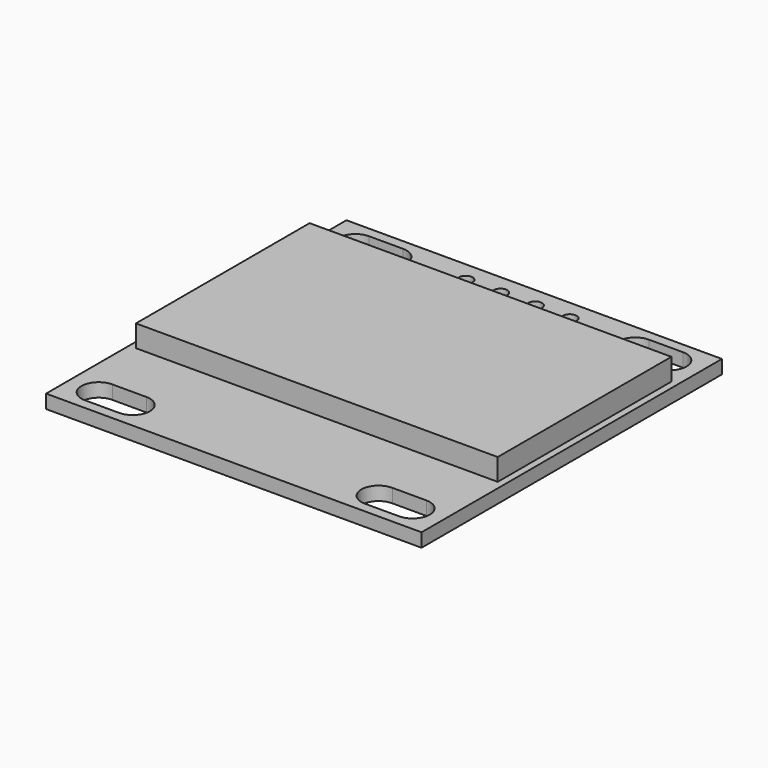
from build123d import *

# Parameters (mm, degrees)
F0_W           = 27.5
F0_H           = 27.5
F1_DEPTH       = 1
F2_W           = 26.5
F2_H           = 15.9
F3_DEPTH       = 1.6
F4_R           = 0.5
F5_DEPTH       = 1.001
F6_TEXT_SIZE   = 1.057064993
F6_TEXT_SIZE_2 = 0.9030619444
F6_TEXT_SIZE_3 = 1.1489094336
F6_TEXT_SIZE_4 = 1.0123378678
F7_DEPTH       = 0.1


# Not quite as in the source:
# - Text() gives the source's letters only with a copy of the font that has no kerning and outlines rounded to 1/6400 em; it was checked with that copy


with BuildPart() as f1:
    # F0 (on Top) → F1 (new body)
    with BuildSketch(Plane.XY):
        Rectangle(F0_W, F0_H)
    extrude(amount=F1_DEPTH)

    # F2 (on face) → F3 (join)
    with BuildSketch(Plane.XY.offset(1)):
        with Locations((0, 1.8)):
            Rectangle(F2_W, F2_H)
    extrude(amount=F3_DEPTH)

    # F4 (on face) → F5 (cut, through all)
    with BuildSketch(Plane.XY.offset(1)):
        with BuildLine():
            Line((-11.5, 10.4937249432), (-9, 10.4937249432))
            ThreePointArc((-9, 10.4937249432), (-7.7437249432, 11.75), (-9, 13.0062750568))
            Line((-9, 13.0062750568), (-11.5, 13.0062750568))
            ThreePointArc((-11.5, 13.0062750568), (-12.7562750568, 11.75), (-11.5, 10.4937249432))
        make_face()
        with Locations((-3.81, 12.25)):
            Circle(F4_R)
        with Locations((-1.27, 12.25)):
            Circle(F4_R)
        with Locations((1.27, 12.25)):
            Circle(F4_R)
        with Locations((3.81, 12.25)):
            Circle(F4_R)
        with BuildLine():
            ThreePointArc((9, 13.0062750568), (7.7437249432, 11.75), (9, 10.4937249432))
            Line((9, 10.4937249432), (11.5, 10.4937249432))
            ThreePointArc((11.5, 10.4937249432), (12.7562750568, 11.75), (11.5, 13.0062750568))
            Line((11.5, 13.0062750568), (9, 13.0062750568))
        make_face()
        with BuildLine():
            ThreePointArc((-9, -13.0062750568), (-7.7437249432, -11.75), (-9, -10.4937249432))
            Line((-9, -10.4937249432), (-11.5, -10.4937249432))
            ThreePointArc((-11.5, -10.4937249432), (-12.7562750568, -11.75), (-11.5, -13.0062750568))
            Line((-11.5, -13.0062750568), (-9, -13.0062750568))
        make_face()
        with BuildLine():
            ThreePointArc((9, -10.4937249432), (7.7437249432, -11.75), (9, -13.0062750568))
            Line((9, -13.0062750568), (11.5, -13.0062750568))
            ThreePointArc((11.5, -13.0062750568), (12.7562750568, -11.75), (11.5, -10.4937249432))
            Line((11.5, -10.4937249432), (9, -10.4937249432))
        make_face()
    extrude(amount=-F5_DEPTH, mode=Mode.SUBTRACT)

    # F6 (on face) → F7 (cut)
    with BuildSketch(Plane.XY.offset(1)):
        with Locations((-4.6618625317, 10.6308086258)):
            Text('VCC', F6_TEXT_SIZE, font='Open Sans', text_align=(TextAlign.LEFT, TextAlign.BOTTOM))
        with Locations((-2.1963005977, 10.7280638144)):
            Text('GND', F6_TEXT_SIZE_2, font='Open Sans', text_align=(TextAlign.LEFT, TextAlign.BOTTOM))
        with Locations((0.2740490817, 10.6351592031)):
            Text('SCL', F6_TEXT_SIZE_3, font='Open Sans', text_align=(TextAlign.LEFT, TextAlign.BOTTOM))
        with Locations((2.891141975, 10.6804623369)):
            Text('SDA', F6_TEXT_SIZE_4, font='Open Sans', text_align=(TextAlign.LEFT, TextAlign.BOTTOM))
    extrude(amount=-F7_DEPTH, mode=Mode.SUBTRACT)


solid = f1.part
